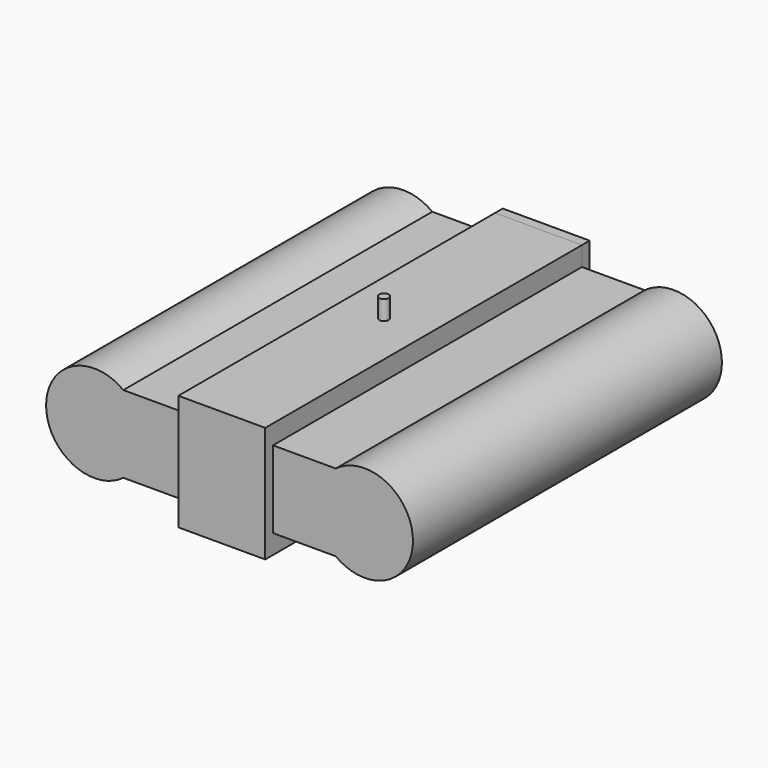
from build123d import *

# Parameters (mm, degrees)
F1_DEPTH   = 100
F3_DEPTH   = 105
F5_DEPTH   = 5
F6_START   = -205
F4_W       = 45
F4_H       = 60
F6_DEPTH   = 5
F7_DEPTH   = 5
F9_D       = 5
F9_DEPTH   = 20
F9_TIP     = 1.5021515476
F9_2_D     = 5
F9_2_DEPTH = 20
F9_2_TIP   = 1.5021515476
F10_R      = 2.5
F11_DEPTH  = 10


with BuildPart() as f1:
    # F0 (on Front) → F1 (new body, symmetric)
    with BuildSketch(Plane.XZ):
        with BuildLine():
            ThreePointArc((55, -20), (81.1803398875, -22.360679775), (95, 0))
            ThreePointArc((95, 0), (81.1803398875, 22.360679775), (55, 20))
            Line((55, 20), (70, 20))
            Line((70, 20), (70, -20))
            Line((70, -20), (55, -20))
        make_face()
        with BuildLine():
            Line((70, 20), (55, 20))
            ThreePointArc((55, 20), (45, 0), (55, -20))
            Line((55, -20), (70, -20))
            Line((70, -20), (70, 20))
        make_face()
        with BuildLine():
            ThreePointArc((55, -20), (45, 0), (55, 20))
            Line((55, 20), (15, 20))
            ThreePointArc((15, 20), (22.360679775, 11.1803398875), (25, 0))
            ThreePointArc((25, 0), (22.360679775, -11.1803398875), (15, -20))
            Line((15, -20), (55, -20))
        make_face()
        with BuildLine():
            Line((-15, 20), (15, 20))
            ThreePointArc((15, 20), (0, 25), (-15, 20))
        make_face()
        with BuildLine():
            ThreePointArc((25, 0), (22.360679775, 11.1803398875), (15, 20))
            Line((15, 20), (-15, 20))
            ThreePointArc((-15, 20), (-25, 0), (-15, -20))
            Line((-15, -20), (15, -20))
            ThreePointArc((15, -20), (22.360679775, -11.1803398875), (25, 0))
        make_face()
        with BuildLine():
            ThreePointArc((-15, -20), (0, -25), (15, -20))
            Line((15, -20), (-15, -20))
        make_face()
        with BuildLine():
            ThreePointArc((-15, -20), (-25, 0), (-15, 20))
            Line((-15, 20), (-55, 20))
            ThreePointArc((-55, 20), (-47.639320225, 11.1803398875), (-45, 0))
            ThreePointArc((-45, 0), (-47.639320225, -11.1803398875), (-55, -20))
            Line((-55, -20), (-15, -20))
        make_face()
        with BuildLine():
            Line((-70, 20), (-55, 20))
            ThreePointArc((-55, 20), (-95, 0), (-55, -20))
            Line((-55, -20), (-70, -20))
            Line((-70, -20), (-70, 20))
        make_face()
        with BuildLine():
            ThreePointArc((-45, 0), (-47.639320225, 11.1803398875), (-55, 20))
            Line((-55, 20), (-70, 20))
            Line((-70, 20), (-70, -20))
            Line((-70, -20), (-55, -20))
            ThreePointArc((-55, -20), (-47.639320225, -11.1803398875), (-45, 0))
        make_face()
    extrude(amount=F1_DEPTH, both=True)


with BuildPart() as f3:
    # F2 (on Front) → F3 (new body, symmetric)
    with BuildSketch(Plane.XZ):
        with BuildLine():
            Line((15, 20), (22.5, 20))
            Line((22.5, 20), (22.5, 30))
            Line((22.5, 30), (-22.5, 30))
            Line((-22.5, 30), (-22.5, 20))
            Line((-22.5, 20), (-15, 20))
            ThreePointArc((-15, 20), (0, 25), (15, 20))
        make_face()
    extrude(amount=F3_DEPTH, both=True)



with BuildPart() as f3b:
    # F2 (on Front) → F3, piece 2 (new body, symmetric)
    with BuildSketch(Plane.XZ):
        with BuildLine():
            Line((22.5, -30), (22.5, -20))
            Line((22.5, -20), (15, -20))
            ThreePointArc((15, -20), (0, -25), (-15, -20))
            Line((-15, -20), (-22.5, -20))
            Line((-22.5, -20), (-22.5, -30))
            Line((-22.5, -30), (22.5, -30))
        make_face()
    extrude(amount=F3_DEPTH, both=True)


with BuildPart() as f3_1:
    add(f3.part)

    add(f3b.part)  # F5 merges F3b
    # F4 (on face) → F5 (join)
    with BuildSketch(Plane.XZ.offset(105)):
        with BuildLine():
            Line((-15, 20), (-22.5, 20))
            Line((-22.5, 20), (-22.5, -30))
            Line((-22.5, -30), (22.5, -30))
            Line((22.5, -30), (22.5, 20))
            Line((22.5, 20), (15, 20))
            ThreePointArc((15, 20), (0, 25), (-15, 20))
        make_face()
    extrude(amount=-F5_DEPTH)

    # F7 (cut): faces of the model
    f7_faces = [f3_1.faces().sort_by_distance(p)[0] for p in [
        (0, 105, 25.8760623382),
        (0, 105, -25.8760623382),
    ]]
    extrude(f7_faces, amount=-F7_DEPTH, mode=Mode.SUBTRACT)

    # F9
    with Locations(Plane(origin=(0, 105, 0), x_dir=(-1, 0, 0), z_dir=(0, 1, 0))):
        with Locations((-17.5, -25), (17.5, 25)):
            Hole(F9_D / 2, depth=F9_DEPTH)
            with Locations((0, 0, -(F9_DEPTH + F9_TIP / 2))):  # 118° drill point
                Cone(0, F9_D / 2, F9_TIP, mode=Mode.SUBTRACT)

    # F10 (on face) → F11 (join)
    with BuildSketch(Plane.XY.offset(30)):
        Circle(F10_R)
    extrude(amount=F11_DEPTH)


with BuildPart() as f6:
    # F4 (on face) → F6 (new body)
    with BuildSketch(Plane.XZ.offset(105).offset(F6_START)):
        Rectangle(F4_W, F4_H)
    extrude(amount=-F6_DEPTH)

    # F9#2
    with Locations(Plane(origin=(0, 105, 0), x_dir=(-1, 0, 0), z_dir=(0, 1, 0))):
        with Locations((-17.5, -25), (17.5, 25)):
            Hole(F9_2_D / 2, depth=F9_2_DEPTH)
            with Locations((0, 0, -(F9_2_DEPTH + F9_2_TIP / 2))):  # 118° drill point
                Cone(0, F9_2_D / 2, F9_2_TIP, mode=Mode.SUBTRACT)


solid = Compound([f1.part, f3_1.part, f6.part])
